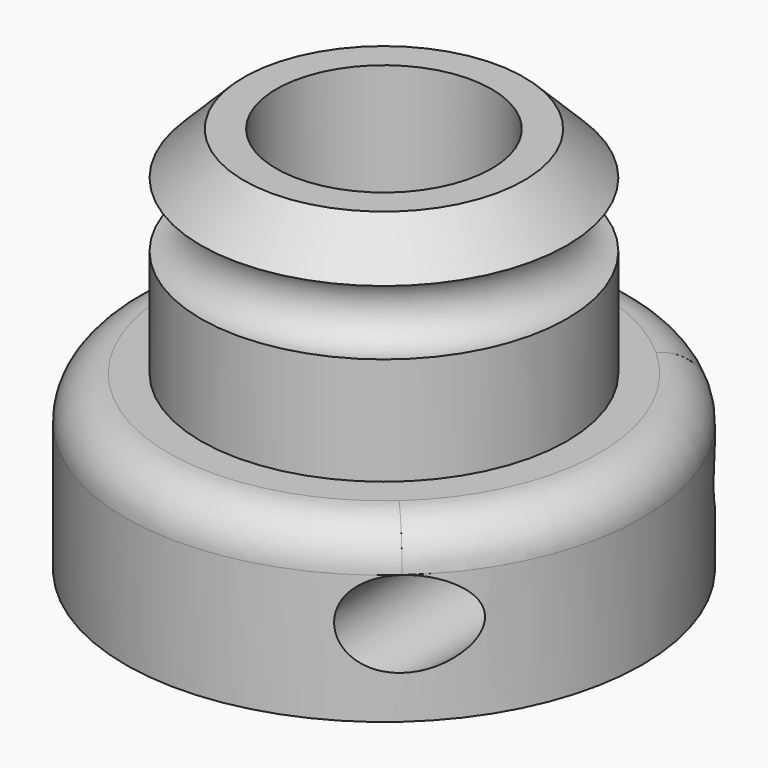
from build123d import *

# Parameters (mm, degrees)
F2_SIZE        = 1.99999
F3_R           = 5
F4_DEPTH       = 6
F5_R           = 12
F6_DEPTH       = 8
F7_R           = 3
F8_DEPTH       = 12
F9_R           = 2
F10_DEPTH      = 12.001
F10_DEPTH_BACK = 12.001
F11_R          = 2


# Not quite as in the source:
# - a fillet or chamfer is up to 0.001 mm smaller than in the source, because OpenCascade refuses the exact size


with BuildPart() as f1:
    # F0 (on Right) → F1 (revolve)
    with BuildSketch(Plane.YZ):
        with BuildLine():
            Line((-8.5, 0), (0, 0))
            Line((0, 0), (0, 10))
            Line((0, 10), (-8.5, 10))
            Line((-8.5, 10), (-8.5, 8))
            ThreePointArc((-8.5, 8), (-7, 6.5), (-8.5, 5))
            Line((-8.5, 5), (-8.5, 0))
        make_face()
    revolve(axis=Axis((0, 0, 5), (0, 0, -1)))

    # F2 (size 2 in the source; OpenCascade refuses exactly that, so slightly less here)
    f2_edges = [f1.edges().sort_by_distance(p)[0] for p in [
        (0, 8.5, 10),
    ]]
    chamfer(f2_edges, length=F2_SIZE)

    # F3 (on face) → F4 (cut)
    with BuildSketch(Plane.XY.offset(10)):
        Circle(F3_R)
    extrude(amount=-F4_DEPTH, mode=Mode.SUBTRACT)

    # F5 (on face) → F6 (join)
    with BuildSketch(Plane(origin=(0, 0, 0), x_dir=(1, 0, 0), z_dir=(0, 0, -1))):
        Circle(F5_R)
    extrude(amount=F6_DEPTH)

    # F7 (on face) → F8 (cut, through all)
    with BuildSketch(Plane.XY.offset(4)):
        Circle(F7_R)
    extrude(amount=-F8_DEPTH, mode=Mode.SUBTRACT)

    # F9 (on Front) → F10 (cut, two sides)
    with BuildSketch(Plane.XZ) as f10_sk:
        with Locations((8, -4)):
            Circle(F9_R)
    extrude(amount=-F10_DEPTH, mode=Mode.SUBTRACT)
    extrude(f10_sk.sketch, amount=F10_DEPTH_BACK, mode=Mode.SUBTRACT)

    # F11
    f11_edges = [f1.edges().sort_by_distance(p)[0] for p in [
        (-12, 0, 0),
    ]]
    fillet(f11_edges, radius=F11_R)


solid = f1.part
